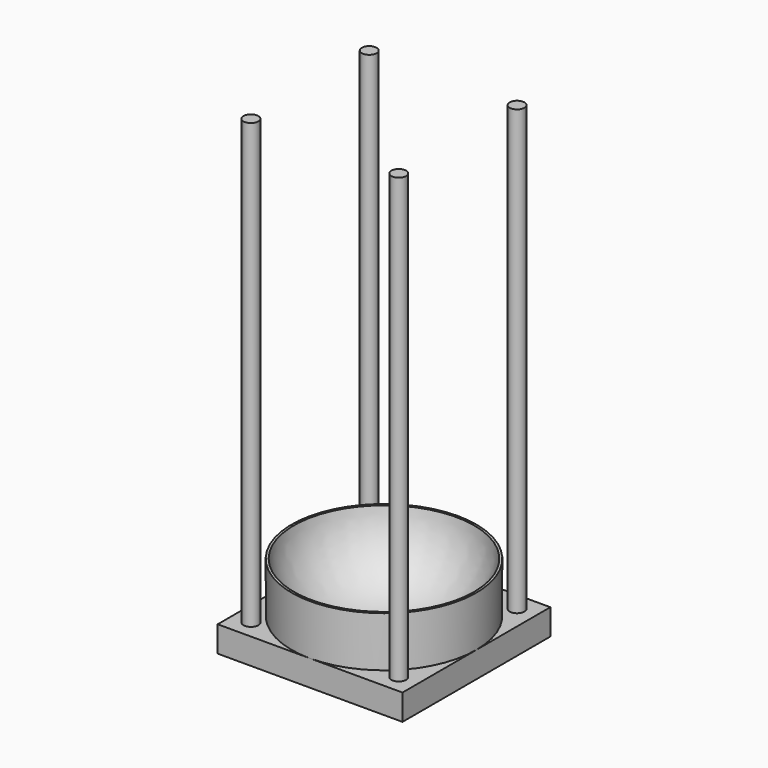
from build123d import *
from build123d import SkipClean  # not in build123d's __all__

# Parameters (mm, degrees)
F0_W     = 63.5
F0_H     = 63.5
F1_DEPTH = 8.89
F2_R     = 2.54
F3_DEPTH = 152.4
F5_DEPTH = 2.032
F6_DEPTH = 15.24
F7_R     = 30.9575720053
F8_DEPTH = 2.54
F9_DEPTH = 20.32


# Not quite as in the source:
# - a fillet or chamfer that OpenCascade refuses, or shapes differently, is made with other operations: its cross-section is extruded or revolved along the edge and cut away or added
# - after a boolean that leaves OpenCascade's solid faulty, fix() repairs it


with BuildPart() as f1:
    # F0 (on Top) → F1 (new body)
    with BuildSketch(Plane.XY):
        Rectangle(F0_W, F0_H)
    extrude(amount=F1_DEPTH)

    # F2 (on face) → F3 (join)
    with BuildSketch(Plane.XY.offset(8.89)):
        with Locations((-25.4, -25.4)):
            Circle(F2_R)
        with Locations((25.4, -25.4)):
            Circle(F2_R)
        with Locations((25.4, 25.4)):
            Circle(F2_R)
        with Locations((-25.4, 25.4)):
            Circle(F2_R)
    extrude(amount=F3_DEPTH)

    # F4 (on face) → F5 (join)
    with BuildSketch(Plane.XY.offset(8.89)):
        with BuildLine():
            ThreePointArc((-3.8e-08, -31.75), (22.4506402893, -22.4506403161), (31.75, 0))
            ThreePointArc((31.75, 0), (22.4506402996, 22.4506403057), (-8.6e-09, 31.75))
            ThreePointArc((-8.6e-09, 31.75), (-22.4506403095, 22.4506402959), (-31.75, -1.06e-08))
            ThreePointArc((-31.75, -1.06e-08), (-22.4506403123, -22.450640293), (-3.8e-08, -31.75))
        make_face()
    extrude(amount=F5_DEPTH)

    # F6 (add): a face of the model
    f6_faces = [f1.faces().sort_by_distance(p)[0] for p in [
        (0, 0, 10.922),
    ]]
    with SkipClean():  # cleaning this boolean's faces spoils the solid; the shape is the same uncleaned
        extrude(f6_faces, amount=F6_DEPTH)

    # F7 (on face) → F8 (cut)
    with BuildSketch(Plane.XY.offset(26.162)):
        Circle(F7_R)
    extrude(amount=-F8_DEPTH, mode=Mode.SUBTRACT)

    add(f1.part.fix(), mode=Mode.REPLACE)

    # F9 (cut): a face of the model
    f9_faces = [f1.faces().sort_by_distance(p)[0] for p in [
        (0, 0, 23.622),
    ]]
    extrude(f9_faces, amount=-F9_DEPTH, mode=Mode.SUBTRACT)

    # F10: fillet of radius 25.7548302834 on 1 edges, made by hand

    # F10_s1 → F10_t2 (revolve)
    with BuildSketch(Plane.XZ):
        with BuildLine():
            ThreePointArc((30.9575720053, 26.162), (22.5233864988, 9.8491866802), (5.3659475833, 3.302))
            Line((5.3659475833, 3.302), (30.9575720053, 3.302))
            Line((30.9575720053, 3.302), (30.9575720053, 26.162))
        make_face()
    revolve(axis=Axis((0, 0, 3.302), (0, 0, 1)))


solid = f1.part
